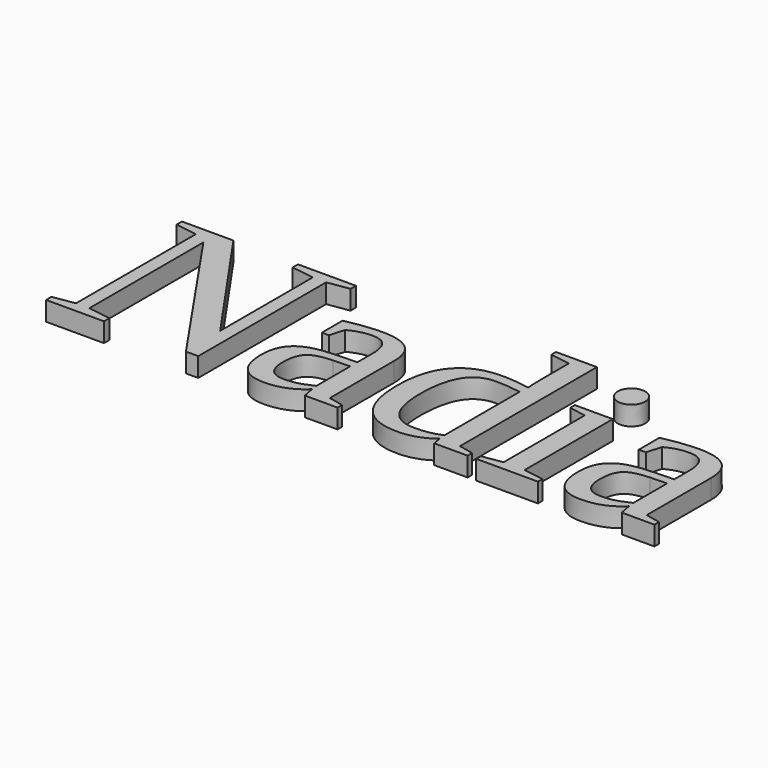
from build123d import *

# Parameters (mm, degrees)
F0_TEXT_SIZE = 51.2647830571
F1_DEPTH     = 3.8


# Not quite as in the source:
# - Text() gives the source's letters only with a copy of the font that has no kerning and outlines rounded to 1/6400 em; it was checked with that copy


with BuildPart() as f1:
    # F0 (on Top) → F1 (new body)
    with BuildSketch(Plane.XY):
        with Locations((-59.4094544649, -18.3726493269)):
            Text('Nadia', F0_TEXT_SIZE, font='Tinos', text_align=(TextAlign.LEFT, TextAlign.BOTTOM))
    extrude(amount=-F1_DEPTH)


solid = f1.part
